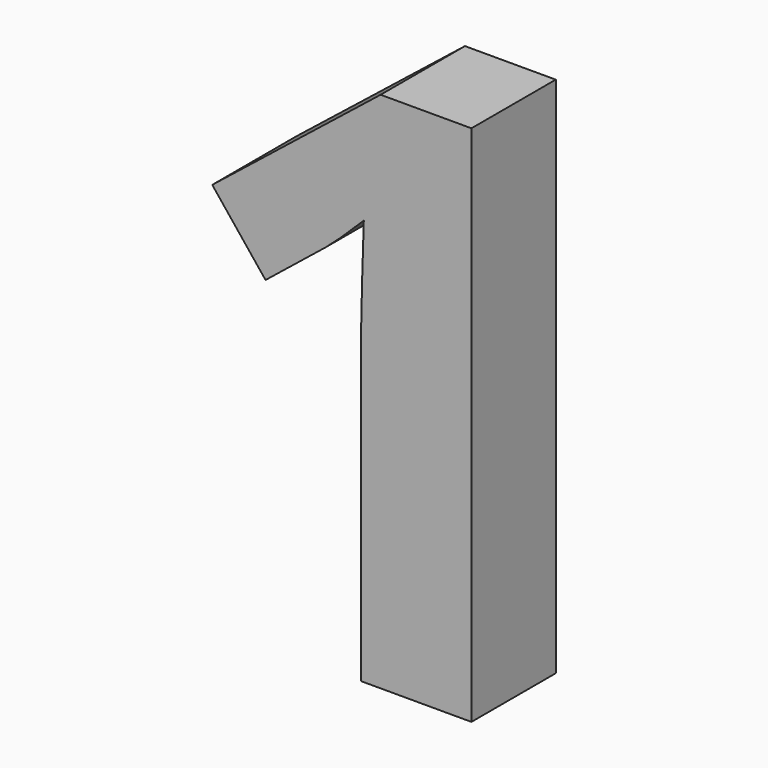
from build123d import *

# Parameters (mm, degrees)
F0_TEXT_SIZE = 35.2777777778
F1_DEPTH     = 5.08


# Not quite as in the source:
# - Text() gives the source's letters only with a copy of the font that has no kerning and outlines rounded to 1/6400 em; it was checked with that copy


with BuildPart() as f1:
    # F0 (on Front) → F1 (new body)
    with BuildSketch(Plane.XZ):
        with Locations((-50.8543135566, 17.2112013967)):
            Text('1', F0_TEXT_SIZE, font='Open Sans', font_style=FontStyle.BOLD, text_align=(TextAlign.LEFT, TextAlign.BOTTOM))
    extrude(amount=F1_DEPTH)


solid = f1.part
